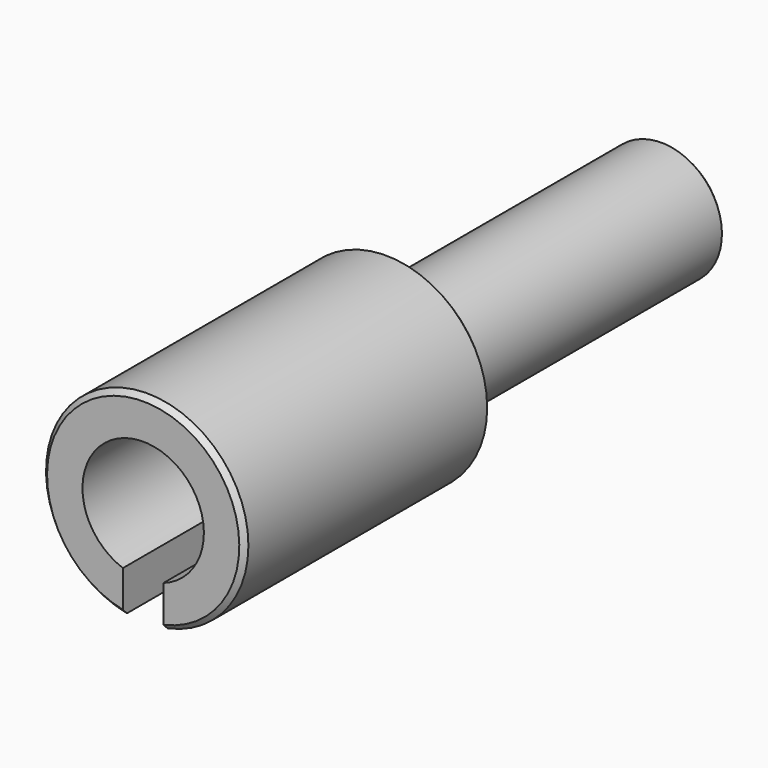
from build123d import *

# Parameters (mm, degrees)
F0_R      = 10
F1_DEPTH  = 30.5
F2_R      = 6
F3_DEPTH  = 20
F4_R      = 6
F5_DEPTH  = 34
F7_W      = 4
F7_H      = 23
F8_DEPTH  = 2.5
F9_R      = 1.9999
F10_W     = 4
F10_H     = 20
F11_DEPTH = 25
F12_R     = 1.9999
F13_SIZE  = 0.5


# Not quite as in the source:
# - a fillet or chamfer is up to 0.001 mm smaller than in the source, because OpenCascade refuses the exact size


with BuildPart() as f1:
    # F0 (on Front) → F1 (new body)
    with BuildSketch(Plane.XZ):
        Circle(F0_R)
    extrude(amount=F1_DEPTH)

    # F2 (on face) → F3 (cut)
    with BuildSketch(Plane.XZ.offset(30.5)):
        Circle(F2_R)
    extrude(amount=-F3_DEPTH, mode=Mode.SUBTRACT)

    # F4 (on face) → F5 (join)
    with BuildSketch(Plane(origin=(0, 0, 0), x_dir=(-1, 0, 0), z_dir=(0, 1, 0))):
        Circle(F4_R)
    extrude(amount=F5_DEPTH)

    # F7 (on offset) → F8 (cut)
    with BuildSketch(Plane.XY.offset(-6)):
        with Locations((0, 22.5)):
            Rectangle(F7_W, F7_H)
    extrude(amount=F8_DEPTH, mode=Mode.SUBTRACT)

    # F9 (radius 2 in the source; OpenCascade refuses exactly that, so slightly less here)
    f9_edges = [f1.edges().sort_by_distance(p)[0] for p in [
        (-2, 11, -4.578427),
        (2, 11, -4.578427),
    ]]
    fillet(f9_edges, radius=F9_R)

    # F10 (on Top) → F11 (cut)
    with BuildSketch(Plane.XY):
        with Locations((0, -20.5)):
            Rectangle(F10_W, F10_H)
    extrude(amount=-F11_DEPTH, mode=Mode.SUBTRACT)

    # F12 (radius 2 in the source; OpenCascade refuses exactly that, so slightly less here)
    f12_edges = [f1.edges().sort_by_distance(p)[0] for p in [
        (2, -10.5, -7.727407),
        (-2, -10.5, -7.727407),
    ]]
    fillet(f12_edges, radius=F12_R)

    # F13
    f13_edges = [f1.edges().sort_by_distance(p)[0] for p in [
        (-10, 0, 0),
        (3.464102, 34, 4.898979),
        (-6.324555, -30.5, 7.745967),
    ]]
    chamfer(f13_edges, length=F13_SIZE)


solid = f1.part
